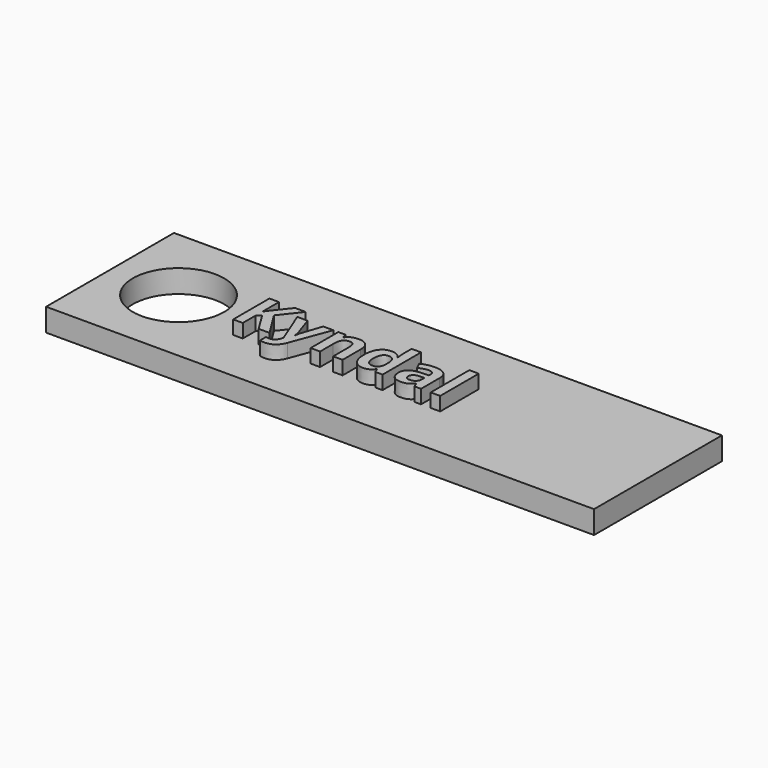
from build123d import *

# Parameters (mm, degrees)
F0_W         = 120
F0_H         = 35
F0_R         = 10
F1_DEPTH     = 5
F2_TEXT_SIZE = 13.8888888889
F4_DEPTH     = 3


# Not quite as in the source:
# - the program builds the solid bodies; features that only make, move or delete a surface that nothing else refers to are left out
# - Text() gives the source's letters only with a copy of the font that has no kerning and outlines rounded to 1/6400 em; it was checked with that copy


with BuildPart() as f1:
    # F0 (on Top) → F1 (new body)
    with BuildSketch(Plane.XY):
        Rectangle(F0_W, F0_H)
        with Locations((-45, 0)):
            Circle(F0_R, mode=Mode.SUBTRACT)
    extrude(amount=-F1_DEPTH)

    # F2 (on face) → F4 (join)
    with BuildSketch(Plane.XY):
        with Locations((-29.7304219025, -5.6863330561)):
            Text('Kyndal', F2_TEXT_SIZE, font='Open Sans', font_style=FontStyle.BOLD, text_align=(TextAlign.LEFT, TextAlign.BOTTOM))
    extrude(amount=F4_DEPTH)


solid = f1.part
